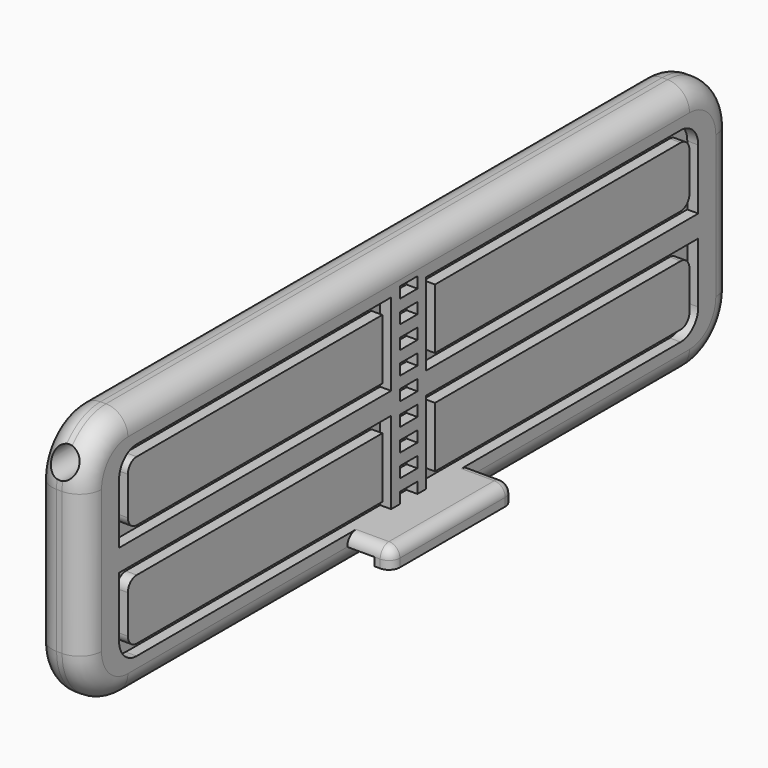
from build123d import *

# Parameters (mm, degrees)
F1_DEPTH     = 4.5
F2_R         = 1.225
F3_DEPTH     = 74
F4_T1_DEPTH  = 64
F4_T3_DEPTH  = 13
F4_T6_ANGLE  = 90
F4_T8_ANGLE  = 90
F4_T10_ANGLE = 90
F4_T12_ANGLE = 90
F4_T14_ANGLE = 90
F4_T16_ANGLE = 90
F4_T18_ANGLE = 90
F4_T20_ANGLE = 90
F6_DEPTH     = 1
F7_W         = 2
F7_H         = 1
F8_DEPTH     = 1
F10_DEPTH    = 1
F11_W        = 14
F11_H        = 1
F12_DEPTH    = 4
F13_W        = 1.5
F13_H        = 14
F14_DEPTH    = 0.75
F15_R        = 0.99999


# Not quite as in the source:
# - a fillet or chamfer that OpenCascade refuses, or shapes differently, is made with other operations: its cross-section is extruded or revolved along the edge and cut away or added
# - a fillet or chamfer is up to 0.001 mm smaller than in the source, because OpenCascade refuses the exact size


with BuildPart() as f1:
    # F0 (on Right) → F1 (new body)
    with BuildSketch(Plane.YZ):
        with BuildLine():
            ThreePointArc((0, 5), (1.4644660941, 1.4644660941), (5, 0))
            Line((5, 0), (69, 0))
            ThreePointArc((69, 0), (72.5355339059, 1.4644660941), (74, 5))
            Line((74, 5), (74, 18))
            ThreePointArc((74, 18), (72.5355339059, 21.5355339059), (69, 23))
            Line((69, 23), (5, 23))
            ThreePointArc((5, 23), (1.4644660941, 21.5355339059), (0, 18))
            Line((0, 18), (0, 5))
        make_face()
    extrude(amount=F1_DEPTH)

    # F2 (on face) → F3 (cut, through all)
    with BuildSketch(Plane(origin=(0, 74, 0), x_dir=(-1, 0, 0), z_dir=(0, 1, 0))):
        with Locations((-2.25, 20)):
            Circle(F2_R)
    extrude(amount=-F3_DEPTH, mode=Mode.SUBTRACT)

    # F4: fillet of radius 2 on 16 edges, made by hand

    # F4_s2 → F4_t1 (cut)
    with BuildSketch(Plane.XZ.offset(-69)):
        with BuildLine():
            ThreePointArc((0, 21), (0.5857864376, 22.4142135624), (2, 23))
            Line((2, 23), (0, 23))
            Line((0, 23), (0, 21))
        make_face()
        with BuildLine():
            ThreePointArc((4.5, 21), (3.9142135624, 22.4142135624), (2.5, 23))
            Line((2.5, 23), (4.5, 23))
            Line((4.5, 23), (4.5, 21))
        make_face()
        with BuildLine():
            ThreePointArc((2, 0), (0.5857864376, 0.5857864376), (0, 2))
            Line((0, 2), (0, 0))
            Line((0, 0), (2, 0))
        make_face()
        with BuildLine():
            ThreePointArc((2.5, 0), (3.9142135624, 0.5857864376), (4.5, 2))
            Line((4.5, 2), (4.5, 0))
            Line((4.5, 0), (2.5, 0))
        make_face()
    extrude(amount=F4_T1_DEPTH, mode=Mode.SUBTRACT)

    # F4_s4 → F4_t3 (cut)
    with BuildSketch(Plane.XY.offset(5)):
        with BuildLine():
            ThreePointArc((2, 0), (0.5857864376, 0.5857864376), (0, 2))
            Line((0, 2), (0, 0))
            Line((0, 0), (2, 0))
        make_face()
        with BuildLine():
            ThreePointArc((2.5, 0), (3.9142135624, 0.5857864376), (4.5, 2))
            Line((4.5, 2), (4.5, 0))
            Line((4.5, 0), (2.5, 0))
        make_face()
        with BuildLine():
            ThreePointArc((0, 72), (0.5857864376, 73.4142135624), (2, 74))
            Line((2, 74), (0, 74))
            Line((0, 74), (0, 72))
        make_face()
        with BuildLine():
            ThreePointArc((4.5, 72), (3.9142135624, 73.4142135624), (2.5, 74))
            Line((2.5, 74), (4.5, 74))
            Line((4.5, 74), (4.5, 72))
        make_face()
    extrude(amount=F4_T3_DEPTH, mode=Mode.SUBTRACT)

    # F4_s5 → F4_t6 (revolve, cut)
    with BuildSketch(Plane.XY.offset(5)):
        with BuildLine():
            ThreePointArc((2, 0), (0.5857864376, 0.5857864376), (0, 2))
            Line((0, 2), (0, 0))
            Line((0, 0), (2, 0))
        make_face()
    revolve(axis=Axis((0, 5, 5), (1, 0, 0)), revolution_arc=F4_T6_ANGLE, mode=Mode.SUBTRACT)

    # F4_s7 → F4_t8 (revolve, cut)
    with BuildSketch(Plane.XY.offset(5)):
        with BuildLine():
            ThreePointArc((2.5, 0), (3.9142135624, 0.5857864376), (4.5, 2))
            Line((4.5, 2), (4.5, 0))
            Line((4.5, 0), (2.5, 0))
        make_face()
    revolve(axis=Axis((4.5, 5, 5), (1, 0, 0)), revolution_arc=F4_T8_ANGLE, mode=Mode.SUBTRACT)

    # F4_s9 → F4_t10 (revolve, cut)
    with BuildSketch(Plane.XZ.offset(-69)):
        with BuildLine():
            ThreePointArc((0, 2), (0.5857864376, 0.5857864376), (2, 0))
            Line((2, 0), (0, 0))
            Line((0, 0), (0, 2))
        make_face()
    revolve(axis=Axis((0, 69, 5), (1, 0, 0)), revolution_arc=F4_T10_ANGLE, mode=Mode.SUBTRACT)

    # F4_s11 → F4_t12 (revolve, cut)
    with BuildSketch(Plane.XY.offset(18)):
        with BuildLine():
            ThreePointArc((0, 72), (0.5857864376, 73.4142135624), (2, 74))
            Line((2, 74), (0, 74))
            Line((0, 74), (0, 72))
        make_face()
    revolve(axis=Axis((0, 69, 18), (1, 0, 0)), revolution_arc=F4_T12_ANGLE, mode=Mode.SUBTRACT)

    # F4_s13 → F4_t14 (revolve, cut)
    with BuildSketch(Plane.XZ.offset(-5)):
        with BuildLine():
            ThreePointArc((0, 21), (0.5857864376, 22.4142135624), (2, 23))
            Line((2, 23), (0, 23))
            Line((0, 23), (0, 21))
        make_face()
    revolve(axis=Axis((0, 5, 18), (1, 0, 0)), revolution_arc=F4_T14_ANGLE, mode=Mode.SUBTRACT)

    # F4_s15 → F4_t16 (revolve, cut)
    with BuildSketch(Plane.XZ.offset(-69)):
        with BuildLine():
            ThreePointArc((4.5, 2), (3.9142135624, 0.5857864376), (2.5, 0))
            Line((2.5, 0), (4.5, 0))
            Line((4.5, 0), (4.5, 2))
        make_face()
    revolve(axis=Axis((4.5, 69, 5), (1, 0, 0)), revolution_arc=F4_T16_ANGLE, mode=Mode.SUBTRACT)

    # F4_s17 → F4_t18 (revolve, cut)
    with BuildSketch(Plane.XY.offset(18)):
        with BuildLine():
            ThreePointArc((4.5, 72), (3.9142135624, 73.4142135624), (2.5, 74))
            Line((2.5, 74), (4.5, 74))
            Line((4.5, 74), (4.5, 72))
        make_face()
    revolve(axis=Axis((4.5, 69, 18), (1, 0, 0)), revolution_arc=F4_T18_ANGLE, mode=Mode.SUBTRACT)

    # F4_s19 → F4_t20 (revolve, cut)
    with BuildSketch(Plane.XZ.offset(-5)):
        with BuildLine():
            ThreePointArc((4.5, 21), (3.9142135624, 22.4142135624), (2.5, 23))
            Line((2.5, 23), (4.5, 23))
            Line((4.5, 23), (4.5, 21))
        make_face()
    revolve(axis=Axis((4.5, 5, 18), (1, 0, 0)), revolution_arc=F4_T20_ANGLE, mode=Mode.SUBTRACT)

    # F5 (on face) → F6 (cut)
    with BuildSketch(Plane.YZ.offset(4.5)):
        with BuildLine():
            Line((35, 20), (6, 20))
            ThreePointArc((6, 20), (4.5857864376, 19.4142135624), (4, 18))
            Line((4, 18), (4, 12.5))
            Line((4, 12.5), (35, 12.5))
            Line((35, 12.5), (35, 20))
        make_face()
        with BuildLine():
            ThreePointArc((4, 5), (4.5857864376, 3.5857864376), (6, 3))
            Line((6, 3), (35, 3))
            Line((35, 3), (35, 10.5))
            Line((35, 10.5), (4, 10.5))
            Line((4, 10.5), (4, 5))
        make_face()
        with BuildLine():
            Line((68, 20), (39, 20))
            Line((39, 20), (39, 12.5))
            Line((39, 12.5), (70, 12.5))
            Line((70, 12.5), (70, 18))
            ThreePointArc((70, 18), (69.4142135624, 19.4142135624), (68, 20))
        make_face()
        with BuildLine():
            Line((39, 10.5), (39, 3))
            Line((39, 3), (68, 3))
            ThreePointArc((68, 3), (69.4142135624, 3.5857864376), (70, 5))
            Line((70, 5), (70, 10.5))
            Line((70, 10.5), (39, 10.5))
        make_face()
    extrude(amount=-F6_DEPTH, mode=Mode.SUBTRACT)

    # F7 (on face) → F8 (cut)
    with BuildSketch(Plane.YZ.offset(4.5)):
        with Locations((37, 3.5)):
            Rectangle(F7_W, F7_H)
        with Locations((37, 5.56)):
            Rectangle(F7_W, F7_H)
        with Locations((37, 7.62)):
            Rectangle(F7_W, F7_H)
        with Locations((37, 9.68)):
            Rectangle(F7_W, F7_H)
        with Locations((37, 11.74)):
            Rectangle(F7_W, F7_H)
        with Locations((37, 13.8)):
            Rectangle(F7_W, F7_H)
        with Locations((37, 15.86)):
            Rectangle(F7_W, F7_H)
        with Locations((37, 17.92)):
            Rectangle(F7_W, F7_H)
        with Locations((37, 19.98)):
            Rectangle(F7_W, F7_H)
    extrude(amount=-F8_DEPTH, mode=Mode.SUBTRACT)

    # F9 (on face) → F10 (join)
    with BuildSketch(Plane.YZ.offset(3.5)):
        with BuildLine():
            ThreePointArc((5, 5), (5.2928932188, 4.2928932188), (6, 4))
            Line((6, 4), (34, 4))
            Line((34, 4), (34, 9.5))
            Line((34, 9.5), (6, 9.5))
            ThreePointArc((6, 9.5), (5.2928932188, 9.2071067812), (5, 8.5))
            Line((5, 8.5), (5, 5))
        make_face()
        with BuildLine():
            Line((34, 19), (6, 19))
            ThreePointArc((6, 19), (5.2928932188, 18.7071067812), (5, 18))
            Line((5, 18), (5, 14.5))
            ThreePointArc((5, 14.5), (5.2928932188, 13.7928932188), (6, 13.5))
            Line((6, 13.5), (34, 13.5))
            Line((34, 13.5), (34, 19))
        make_face()
        with BuildLine():
            ThreePointArc((69, 8.5), (68.7071067812, 9.2071067812), (68, 9.5))
            Line((68, 9.5), (40, 9.5))
            Line((40, 9.5), (40, 4))
            Line((40, 4), (68, 4))
            ThreePointArc((68, 4), (68.7071067812, 4.2928932188), (69, 5))
            Line((69, 5), (69, 8.5))
        make_face()
        with BuildLine():
            ThreePointArc((68, 13.5), (68.7071067812, 13.7928932188), (69, 14.5))
            Line((69, 14.5), (69, 18))
            ThreePointArc((69, 18), (68.7071067812, 18.7071067812), (68, 19))
            Line((68, 19), (40, 19))
            Line((40, 19), (40, 13.5))
            Line((40, 13.5), (68, 13.5))
        make_face()
    extrude(amount=F10_DEPTH)

    # F11 (on face) → F12 (join)
    with BuildSketch(Plane.YZ.offset(4.5)):
        with Locations((37, 2.5)):
            Rectangle(F11_W, F11_H)
    extrude(amount=F12_DEPTH)

    # F13 (on face) → F14 (join)
    with BuildSketch(Plane(origin=(0, 0, 2), x_dir=(1, 0, 0), z_dir=(0, 0, -1))):
        with Locations((7.75, -37)):
            Rectangle(F13_W, F13_H)
    extrude(amount=F14_DEPTH)

    # F15 (radius 1 in the source; OpenCascade refuses exactly that, so slightly less here)
    f15_edges = [f1.edges().sort_by_distance(p)[0] for p in [
        (8.5, 37, 3),
        (6.5, 30, 3),
        (6.5, 44, 3),
        (8.5, 44, 2.125),
        (8.5, 30, 2.125),
    ]]
    fillet(f15_edges, radius=F15_R)


solid = f1.part
